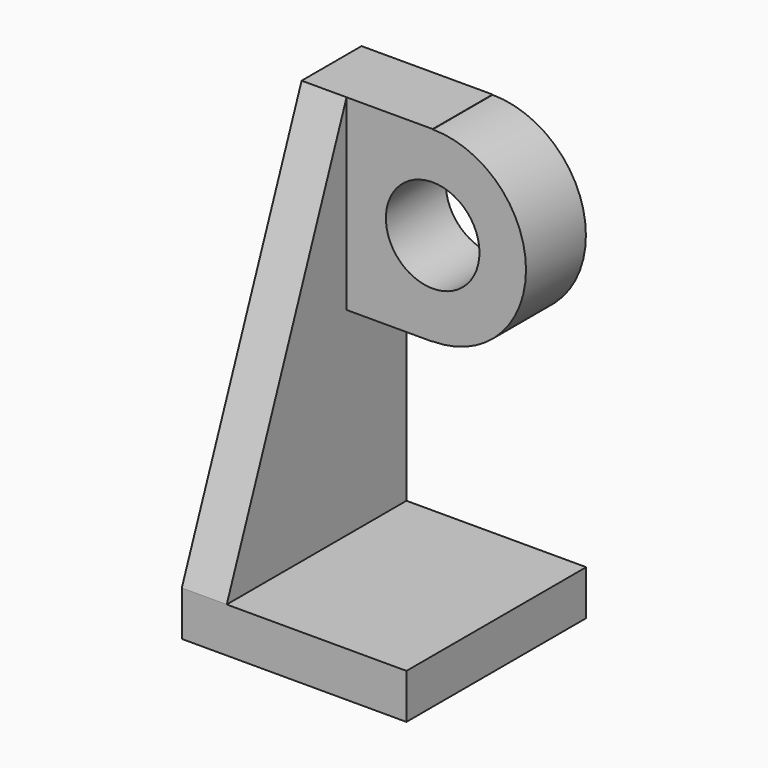
from build123d import *

# Parameters (mm, degrees)
F0_W     = 1524
F0_H     = 1524
F1_DEPTH = 304.8
F3_DEPTH = 304.8
F4_W     = 508
F4_H     = 1270
F5_DEPTH = 584.2
F7_DEPTH = 508
F8_R     = 317.5
F9_DEPTH = 508


with BuildPart() as f1:
    # F0 (on Top) → F1 (new body)
    with BuildSketch(Plane.XY):
        with Locations((601.377745986, 711.8515538871)):
            Rectangle(F0_W, F0_H)
    extrude(amount=F1_DEPTH)

    # F2 (on face) → F3 (join)
    with BuildSketch(Plane(origin=(-160.622254014, 0, 0), x_dir=(0, -1, 0), z_dir=(-1, 0, 0))):
        Polygon((-1473.8515538871, 2921), (-1473.8515538871, 304.8), (50.1484461129, 304.8), (-965.8515538871, 2921), align=None)
    extrude(amount=-F3_DEPTH)

    # F4 (on face) → F5 (join)
    with BuildSketch(Plane.YZ.offset(144.177745986)):
        with Locations((1219.8515538871, 2286)):
            Rectangle(F4_W, F4_H)
    extrude(amount=F5_DEPTH)

    # F6 (on face) → F7 (join)
    with BuildSketch(Plane.XZ.offset(-965.8515538871)):
        with BuildLine():
            ThreePointArc((728.377745986, 1652.952168632), (1176.0101603617, 1838.3675856243), (1361.425577354, 2286))
            ThreePointArc((1361.425577354, 2286), (1176.0101603617, 2733.6324143757), (728.377745986, 2919.047831368))
            Line((728.377745986, 2919.047831368), (728.377745986, 1652.952168632))
        make_face()
    extrude(amount=-F7_DEPTH)

    # F8 (on face) → F9 (cut)
    with BuildSketch(Plane.XZ.offset(-965.8515538871)):
        with Locations((728.377745986, 2286)):
            Circle(F8_R)
    extrude(amount=-F9_DEPTH, mode=Mode.SUBTRACT)


solid = f1.part
